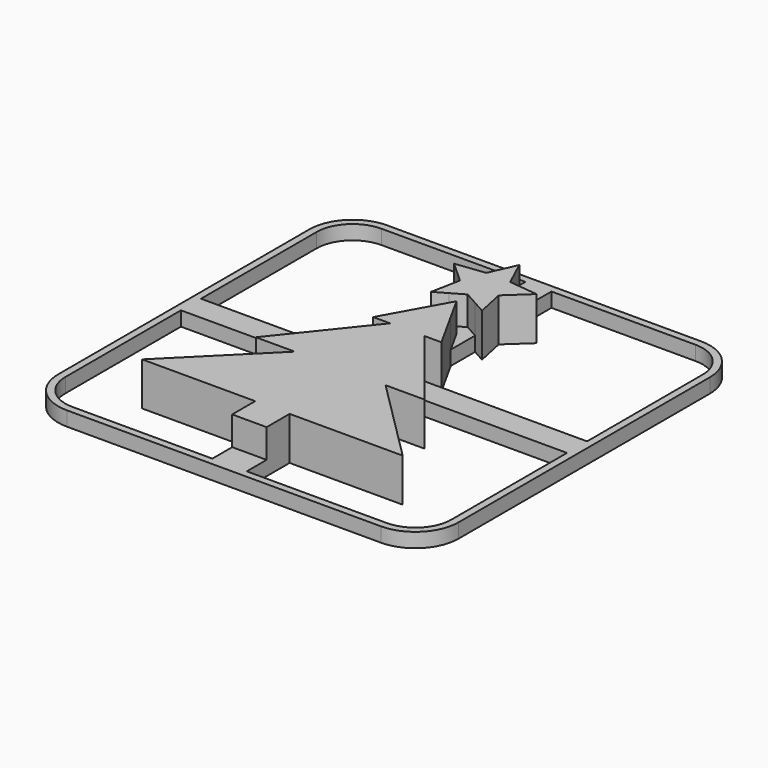
from build123d import *

# Parameters (mm, degrees)
F1_DEPTH = 1
F3_DEPTH = 2
F4_DEPTH = 25


# Not quite as in the source:
# - a feature names something its author has since deleted; it is built from what else it names


with BuildPart() as f1:
    # F0 (on Top) → F1 (new body)
    with BuildSketch(Plane.XY):
        with BuildLine():
            ThreePointArc((-10.9, 13.9), (-13.0213203436, 13.0213203436), (-13.9, 10.9))
            Line((-13.9, 10.9), (-13.9, -10.9))
            ThreePointArc((-13.9, -10.9), (-13.0213203436, -13.0213203436), (-10.9, -13.9))
            Line((-10.9, -13.9), (10.9, -13.9))
            ThreePointArc((10.9, -13.9), (13.0213203436, -13.0213203436), (13.9, -10.9))
            Line((13.9, -10.9), (13.9, 10.9))
            ThreePointArc((13.9, 10.9), (13.0213203436, 13.0213203436), (10.9, 13.9))
            Line((10.9, 13.9), (-10.9, 13.9))
        make_face()
    extrude(amount=F1_DEPTH)

    # F2 (on face) → F3 (join)
    with BuildSketch(Plane.XY.offset(1)):
        Polygon((-0.8220698815, 9.9003828379), (-0.9031134541, 9.8906987285), (-2.8628115953, 9.6565292491), (-1.3706095432, 8.3073079855), (-1.7693148693, 6.2910923774), (-0.9031134541, 6.7887921262), (-0.0250134015, 7.2933285631), (0.9031134541, 6.7749159991), (1.7693148693, 6.2910923774), (1.3551504109, 8.2597296685), (2.8628115953, 9.6565292491), (0.9031134541, 9.8666282056), (0.8625424153, 9.8709778209), (0, 11.7364836228), align=None)
        Polygon((-1.1949065374, 2.0178125706), (-2.11299252, 0.8704443462), (2.11299252, 0.8704443462), (1.1949065374, 2.0178125706), (2.3687703069, 2.0178125706), (0.9031134541, 4.6618687775), (0, 6.2910923774), (-0.9324762655, 4.6088980406), (-2.3687703069, 2.0178125706), align=None)
        Polygon((3.5059938878, -0.8704443462), (-3.5059938878, -0.8704443462), (-5.8554494827, -3.8066515699), (-3.1518915202, -3.8066515699), (-9.0449256822, -9.6830716357), (-1.1949065374, -9.6830716357), (-1.1949065374, -11.6795562208), (0, -11.6795562208), (1.1949065374, -11.6795562208), (1.1949065374, -9.6830716357), (9.0449256822, -9.6830716357), (3.1518915202, -3.8066515699), (5.8554494827, -3.8066515699), align=None)
        Polygon((2.11299252, 0.8704443462), (-2.11299252, 0.8704443462), (-3.5059938878, -0.8704443462), (3.5059938878, -0.8704443462), align=None)
    extrude(amount=F3_DEPTH)

    # F2 (on face) → F4 (cut)
    with BuildSketch(Plane.XY.offset(1)):
        with BuildLine():
            ThreePointArc((-10.9, 13.4), (-12.667766953, 12.667766953), (-13.4, 10.9))
            Line((-13.4, 10.9), (-13.4, 0.8704443462))
            Line((-13.4, 0.8704443462), (-2.11299252, 0.8704443462))
            Line((-2.11299252, 0.8704443462), (-1.1949065374, 2.0178125706))
            Line((-1.1949065374, 2.0178125706), (-2.3687703069, 2.0178125706))
            Line((-2.3687703069, 2.0178125706), (-0.9324762655, 4.6088980406))
            Line((-0.9324762655, 4.6088980406), (-0.9031134541, 6.2910923774))
            Line((-0.9031134541, 6.2910923774), (-0.9031134541, 6.7887921262))
            Line((-0.9031134541, 6.7887921262), (-1.7693148693, 6.2910923774))
            Line((-1.7693148693, 6.2910923774), (-1.3706095432, 8.3073079855))
            Line((-1.3706095432, 8.3073079855), (-2.8628115953, 9.6565292491))
            Line((-2.8628115953, 9.6565292491), (-0.9031134541, 9.8906987285))
            Line((-0.9031134541, 9.8906987285), (-0.9031134541, 13.4))
            Line((-0.9031134541, 13.4), (-10.9, 13.4))
        make_face()
        with BuildLine():
            Line((1.1949065374, 2.0178125706), (2.11299252, 0.8704443462))
            Line((2.11299252, 0.8704443462), (13.4, 0.8704443462))
            Line((13.4, 0.8704443462), (13.4, 10.9))
            ThreePointArc((13.4, 10.9), (12.667766953, 12.667766953), (10.9, 13.4))
            Line((10.9, 13.4), (0.9031134541, 13.4))
            Line((0.9031134541, 13.4), (0.9031134541, 9.8666282056))
            Line((0.9031134541, 9.8666282056), (2.8628115953, 9.6565292491))
            Line((2.8628115953, 9.6565292491), (1.3551504109, 8.2597296685))
            Line((1.3551504109, 8.2597296685), (1.7693148693, 6.2910923774))
            Line((1.7693148693, 6.2910923774), (0.9031134541, 6.7749159991))
            Line((0.9031134541, 6.7749159991), (0.9031134541, 6.2910923774))
            Line((0.9031134541, 6.2910923774), (0.9031134541, 4.6618687775))
            Line((0.9031134541, 4.6618687775), (2.3687703069, 2.0178125706))
            Line((2.3687703069, 2.0178125706), (1.1949065374, 2.0178125706))
        make_face()
        with BuildLine():
            Line((-3.5059938878, -0.8704443462), (-13.4, -0.8704443462))
            Line((-13.4, -0.8704443462), (-13.4, -10.9))
            ThreePointArc((-13.4, -10.9), (-12.667766953, -12.667766953), (-10.9, -13.4))
            Line((-10.9, -13.4), (-1.1949065374, -13.4))
            Line((-1.1949065374, -13.4), (-1.1949065374, -11.6795562208))
            Line((-1.1949065374, -11.6795562208), (-1.1949065374, -9.6830716357))
            Line((-1.1949065374, -9.6830716357), (-9.0449256822, -9.6830716357))
            Line((-9.0449256822, -9.6830716357), (-3.1518915202, -3.8066515699))
            Line((-3.1518915202, -3.8066515699), (-5.8554494827, -3.8066515699))
            Line((-5.8554494827, -3.8066515699), (-3.5059938878, -0.8704443462))
        make_face()
        with BuildLine():
            Line((13.4, -0.8704443462), (3.5059938878, -0.8704443462))
            Line((3.5059938878, -0.8704443462), (5.8554494827, -3.8066515699))
            Line((5.8554494827, -3.8066515699), (3.1518915202, -3.8066515699))
            Line((3.1518915202, -3.8066515699), (9.0449256822, -9.6830716357))
            Line((9.0449256822, -9.6830716357), (1.1949065374, -9.6830716357))
            Line((1.1949065374, -9.6830716357), (1.1949065374, -11.6795562208))
            Line((1.1949065374, -11.6795562208), (1.1949065374, -13.4))
            Line((1.1949065374, -13.4), (10.9, -13.4))
            ThreePointArc((10.9, -13.4), (12.667766953, -12.667766953), (13.4, -10.9))
            Line((13.4, -10.9), (13.4, -0.8704443462))
        make_face()
    extrude(amount=-F4_DEPTH, mode=Mode.SUBTRACT)


solid = f1.part
